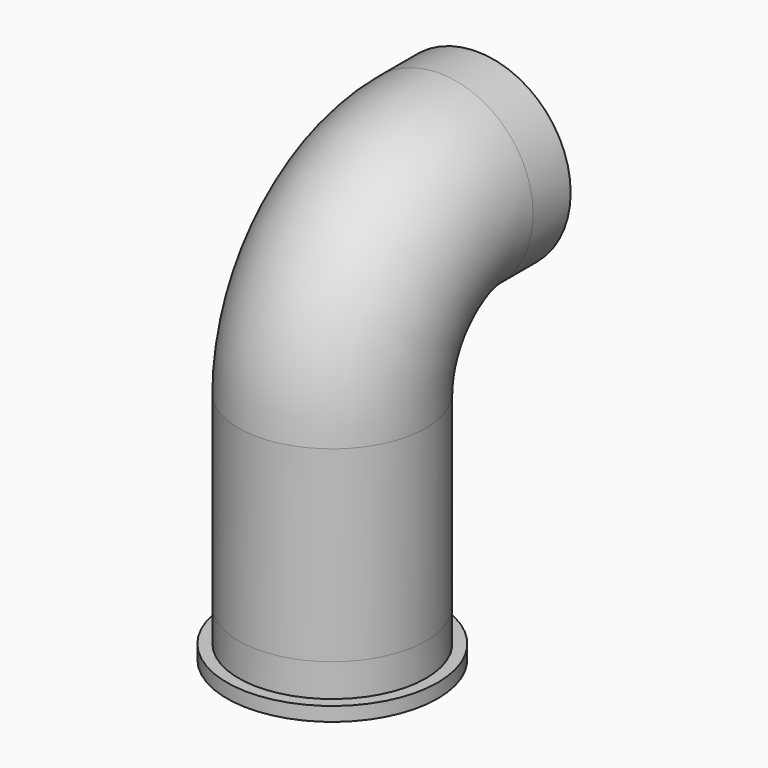
from build123d import *

# Parameters (mm, degrees)
F0_R     = 20
F0_R_2   = 16.5
F3_R     = 20
F3_R_2   = 12.5
F4_DEPTH = 10
F5_R     = 16
F5_R_2   = 12.5
F6_DEPTH = 15
F7_R     = 22.5
F7_R_2   = 20
F8_DEPTH = 3


with BuildPart() as f2:
    # F2: sweep along a path in F1
    with BuildLine(Plane.YZ) as f2_path:
        Line((38.5739039603, 78.5739039603), (28.5739039603, 78.5739039603))
        ThreePointArc((28.5739039603, 78.5739039603), (8.369102705, 70.2048012553), (0, 50))
        Line((0, 50), (0, 0))
    # F0 (on Top) → F2 (sweep)
    with BuildSketch(Plane.XY):
        Circle(F0_R)
        Circle(F0_R_2, mode=Mode.SUBTRACT)
    sweep(path=f2_path.line)


with BuildPart() as f4:
    # F3 (on Top) → F4 (new body)
    with BuildSketch(Plane.XY):
        Circle(F3_R)
        Circle(F3_R_2, mode=Mode.SUBTRACT)
    extrude(amount=F4_DEPTH)

    # F5 (on face) → F6 (join)
    with BuildSketch(Plane.XY.offset(10)):
        Circle(F5_R)
        Circle(F5_R_2, mode=Mode.SUBTRACT)
    extrude(amount=F6_DEPTH)

    # F7 (on Top) → F8 (join)
    with BuildSketch(Plane.XY):
        Circle(F7_R)
        Circle(F7_R_2, mode=Mode.SUBTRACT)
    extrude(amount=F8_DEPTH)


solid = Compound([f2.part, f4.part])
